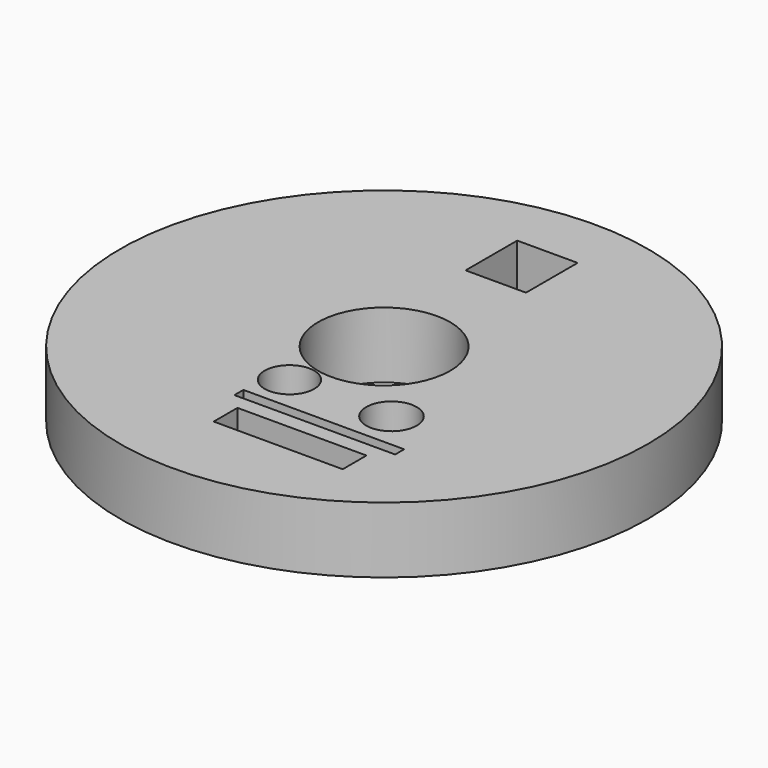
from build123d import *

# Parameters (mm, degrees)
F0_R     = 50.8
F0_R_2   = 4.7623858448
F0_R_3   = 12.7
F0_W     = 24.8306924477
F0_H     = 5.7149995118
F0_W_2   = 30.9398272075
F0_H_2   = 2.1677576005
F0_R_4   = 4.8592779804
F0_W_3   = 11.6270687431
F0_H_3   = 12.4153457582
F1_DEPTH = 6.35


# Not quite as in the source:
# - a length typed as a fraction of an inch, garbled in the dataset ("3 / 203.2 mm" for 3/8 in), is restored


with BuildPart() as f1:
    # F0 (on Top) → F1 (new body, symmetric)
    with BuildSketch(Plane.XY):
        Circle(F0_R)
        with Locations((-4.3355170637, -17.3420701176)):
            Circle(F0_R_2, mode=Mode.SUBTRACT)
        Circle(F0_R_3, mode=Mode.SUBTRACT)
        with Locations((7.6856906526, -32.2207761928)):
            Rectangle(F0_W, F0_H, mode=Mode.SUBTRACT)
        with Locations((7.7842238825, -25.3233611584)):
            Rectangle(F0_W_2, F0_H_2, mode=Mode.SUBTRACT)
        with Locations((15.0699028745, -17.0589182526)):
            Circle(F0_R_4, mode=Mode.SUBTRACT)
        with Locations((-0.0985348597, 33.206121996)):
            Rectangle(F0_W_3, F0_H_3, mode=Mode.SUBTRACT)
    extrude(amount=F1_DEPTH, both=True)


solid = f1.part
